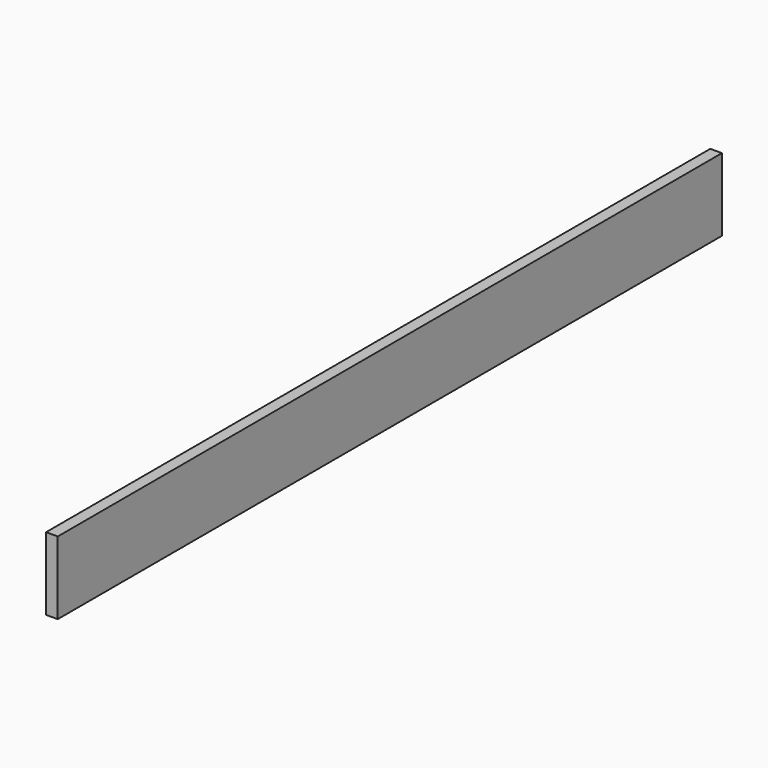
from build123d import *

# Parameters (mm, degrees)
F1_DEPTH = 142.5


# Not quite as in the source:
# - a feature names something its author has since deleted; it is built from what else it names


with BuildPart() as f1:
    # F0 (on Front) → F1 (new body, symmetric)
    with BuildSketch(Plane.XZ):
        Polygon((2, 9.5), (2, 12.5), (-2, 12.5), (-2, -12.5), (2, -12.5), align=None)
    extrude(amount=F1_DEPTH, both=True)


solid = f1.part
